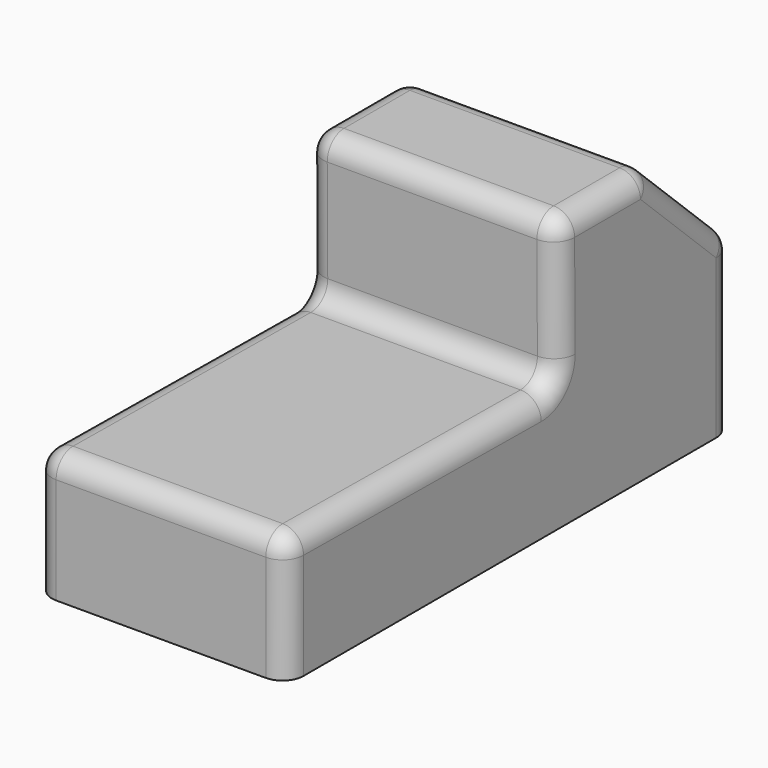
from build123d import *

# Parameters (mm, degrees)
F3_DEPTH  = 30
F4_DEPTH  = 12.5
F5_DEPTH  = 12.5
F6_DEPTH  = 12.5
F7_DEPTH  = 12.5
F8_DEPTH  = 30
F9_R      = 5
F10_T     = -2.5
F2_R      = 4
F2_R_2    = 1.25
F11_DEPTH = 25


with BuildPart() as f3:
    # F0 (on Right) → F3 (new body, symmetric)
    with BuildSketch(Plane.YZ):
        with BuildLine():
            Line((-60.6099627912, 30.3939455835), (-60.6099627912, 0))
            Line((-60.6099627912, 0), (-40.8299627912, 0))
            ThreePointArc((-40.8299627912, 0), (-28.8299627912, 12), (-16.8299627912, 0))
            Line((-16.8299627912, 0), (30.5578776426, 0))
            ThreePointArc((30.5578776426, 0), (41.3865220854, 13.9579662735), (54.3900372088, 2))
            ThreePointArc((54.3900372088, 2), (54.3480034823, 0.9964848766), (54.222196775, 0))
            Line((54.222196775, 0), (72.3900372088, 0))
            Line((72.3900372088, 0), (72.3900372088, 39.934851595))
            Line((72.3900372088, 39.934851595), (46.8496945841, 64.2374157906))
            Line((46.8496945841, 64.2374157906), (20.1869886369, 64.2374157906))
            Line((20.1869886369, 64.2374157906), (20.4051136971, 29.5555796474))
            Line((20.4051136971, 29.5555796474), (-60.6099627912, 30.3939455835))
        make_face()
    extrude(amount=F3_DEPTH, both=True)

    # F0 (on Right) → F4 (join, symmetric)
    with BuildSketch(Plane.YZ):
        with BuildLine():
            Line((-60.6099627912, 30.3939455835), (-60.6099627912, 0))
            Line((-60.6099627912, 0), (-40.8299627912, 0))
            ThreePointArc((-40.8299627912, 0), (-28.8299627912, 12), (-16.8299627912, 0))
            Line((-16.8299627912, 0), (30.5578776426, 0))
            ThreePointArc((30.5578776426, 0), (41.3865220854, 13.9579662735), (54.3900372088, 2))
            ThreePointArc((54.3900372088, 2), (54.3480034823, 0.9964848766), (54.222196775, 0))
            Line((54.222196775, 0), (72.3900372088, 0))
            Line((72.3900372088, 0), (72.3900372088, 39.934851595))
            Line((72.3900372088, 39.934851595), (46.8496945841, 64.2374157906))
            Line((46.8496945841, 64.2374157906), (20.1869886369, 64.2374157906))
            Line((20.1869886369, 64.2374157906), (20.4051136971, 29.5555796474))
            Line((20.4051136971, 29.5555796474), (-60.6099627912, 30.3939455835))
        make_face()
    extrude(amount=F4_DEPTH, both=True)

    # F0 (on Right) → F5 (join, symmetric)
    with BuildSketch(Plane.YZ):
        with BuildLine():
            Line((-60.6099627912, 30.3939455835), (-60.6099627912, 0))
            Line((-60.6099627912, 0), (-40.8299627912, 0))
            ThreePointArc((-40.8299627912, 0), (-28.8299627912, 12), (-16.8299627912, 0))
            Line((-16.8299627912, 0), (30.5578776426, 0))
            ThreePointArc((30.5578776426, 0), (41.3865220854, 13.9579662735), (54.3900372088, 2))
            ThreePointArc((54.3900372088, 2), (54.3480034823, 0.9964848766), (54.222196775, 0))
            Line((54.222196775, 0), (72.3900372088, 0))
            Line((72.3900372088, 0), (72.3900372088, 39.934851595))
            Line((72.3900372088, 39.934851595), (46.8496945841, 64.2374157906))
            Line((46.8496945841, 64.2374157906), (20.1869886369, 64.2374157906))
            Line((20.1869886369, 64.2374157906), (20.4051136971, 29.5555796474))
            Line((20.4051136971, 29.5555796474), (-60.6099627912, 30.3939455835))
        make_face()
    extrude(amount=F5_DEPTH, both=True)

    # F0 (on Right) → F6 (join, symmetric)
    with BuildSketch(Plane.YZ):
        with BuildLine():
            Line((-60.6099627912, 30.3939455835), (-60.6099627912, 0))
            Line((-60.6099627912, 0), (-40.8299627912, 0))
            ThreePointArc((-40.8299627912, 0), (-28.8299627912, 12), (-16.8299627912, 0))
            Line((-16.8299627912, 0), (30.5578776426, 0))
            ThreePointArc((30.5578776426, 0), (41.3865220854, 13.9579662735), (54.3900372088, 2))
            ThreePointArc((54.3900372088, 2), (54.3480034823, 0.9964848766), (54.222196775, 0))
            Line((54.222196775, 0), (72.3900372088, 0))
            Line((72.3900372088, 0), (72.3900372088, 39.934851595))
            Line((72.3900372088, 39.934851595), (46.8496945841, 64.2374157906))
            Line((46.8496945841, 64.2374157906), (20.1869886369, 64.2374157906))
            Line((20.1869886369, 64.2374157906), (20.4051136971, 29.5555796474))
            Line((20.4051136971, 29.5555796474), (-60.6099627912, 30.3939455835))
        make_face()
    extrude(amount=F6_DEPTH, both=True)

    # F0 (on Right) → F7 (join, symmetric)
    with BuildSketch(Plane.YZ):
        with BuildLine():
            Line((-60.6099627912, 30.3939455835), (-60.6099627912, 0))
            Line((-60.6099627912, 0), (-40.8299627912, 0))
            ThreePointArc((-40.8299627912, 0), (-28.8299627912, 12), (-16.8299627912, 0))
            Line((-16.8299627912, 0), (30.5578776426, 0))
            ThreePointArc((30.5578776426, 0), (41.3865220854, 13.9579662735), (54.3900372088, 2))
            ThreePointArc((54.3900372088, 2), (54.3480034823, 0.9964848766), (54.222196775, 0))
            Line((54.222196775, 0), (72.3900372088, 0))
            Line((72.3900372088, 0), (72.3900372088, 39.934851595))
            Line((72.3900372088, 39.934851595), (46.8496945841, 64.2374157906))
            Line((46.8496945841, 64.2374157906), (20.1869886369, 64.2374157906))
            Line((20.1869886369, 64.2374157906), (20.4051136971, 29.5555796474))
            Line((20.4051136971, 29.5555796474), (-60.6099627912, 30.3939455835))
        make_face()
    extrude(amount=F7_DEPTH, both=True)

    # F0 (on Right) → F8 (join, symmetric)
    with BuildSketch(Plane.YZ):
        with BuildLine():
            ThreePointArc((-16.8299627912, 0), (-28.8299627912, 12), (-40.8299627912, 0))
            Line((-40.8299627912, 0), (-16.8299627912, 0))
        make_face()
        with BuildLine():
            ThreePointArc((54.3900372088, 2), (41.3865220854, 13.9579662735), (30.5578776426, 0))
            Line((30.5578776426, 0), (54.222196775, 0))
            ThreePointArc((54.222196775, 0), (54.3480034823, 0.9964848766), (54.3900372088, 2))
        make_face()
    extrude(amount=F8_DEPTH, both=True)

    # F9
    f9_edges = [f3.edges().sort_by_distance(p)[0] for p in [
        (-30, -20.102425, 29.974763),
        (0, -60.609963, 30.393946),
        (30, -20.102425, 29.974763),
        (0, 20.405114, 29.55558),
        (0, 20.186989, 64.237416),
        (-30, 33.518342, 64.237416),
        (0, 46.849695, 64.237416),
        (30, 33.518342, 64.237416),
        (-30, -60.609963, 15.196973),
        (30, -60.609963, 15.196973),
        (-30, 59.619866, 52.086134),
        (-30, 72.390037, 19.967426),
        (0, 72.390037, 39.934852),
        (30, 59.619866, 52.086134),
        (30, 72.390037, 19.967426),
        (30, 20.296051, 46.896498),
        (-30, 20.296051, 46.896498),
    ]]
    fillet(f9_edges, radius=F9_R)

    # F10
    f10_openings = [f3.faces().sort_by_distance(p)[0] for p in [
        (0, 5.890037, 0),
    ]]
    offset(amount=F10_T, openings=f10_openings)

    # F2 (on offset) → F11, piece 2 (join)
    with BuildSketch(Plane.XY.offset(3)):
        with Locations((13, -38.7313138237)):
            Circle(F2_R)
        with Locations((13, -38.7313138237)):
            Circle(F2_R_2, mode=Mode.SUBTRACT)
        with Locations((-13, -38.7313138237)):
            Circle(F2_R)
        with Locations((-13, -38.7313138237)):
            Circle(F2_R_2, mode=Mode.SUBTRACT)
    extrude(amount=F11_DEPTH)


with BuildPart() as f11:
    # F2 (on offset) → F11 (new body)
    with BuildSketch(Plane.XY.offset(3)):
        with Locations((0, 61.2686861763)):
            Circle(F2_R)
        with Locations((0, 61.2686861763)):
            Circle(F2_R_2, mode=Mode.SUBTRACT)
    extrude(amount=F11_DEPTH)


solid = Compound([f3.part, f11.part])
